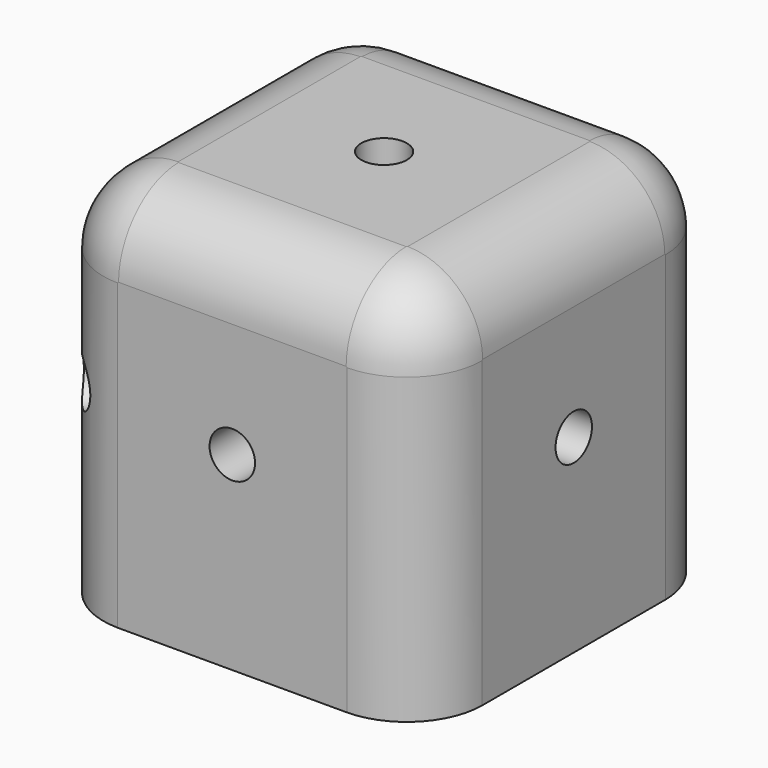
from build123d import *

# Parameters (mm, degrees)
F0_W         = 25
F0_H         = 25
F1_DEPTH     = 12.5
F2_R         = 1.5
F3_DEPTH     = 25
F4_R         = 1.5
F5_DEPTH     = 25.001
F6_R         = 1.5
F7_DEPTH     = 25.001
F8_T1_DEPTH  = 32.5014485681
F8_T3_DEPTH  = 14.9980686292
F8_T5_DEPTH  = 14.9980686292
F8_S9_W      = 5.5015022539
F8_S9_H      = 5.5015022539
F8_T10_DEPTH = 5.501502254
F8_S15_W     = 5.5015022539
F8_S15_H     = 5.5015022539
F8_T16_DEPTH = 5.501502254
F8_S21_W     = 5.5015022539
F8_S21_H     = 5.5015022539
F8_T22_DEPTH = 5.501502254
F8_S27_W     = 5.5015022539
F8_S27_H     = 5.5015022539
F8_T28_DEPTH = 5.501502254
F10_R        = 1.5
F11_DEPTH    = 31.8208051534
F13_R        = 1.5
F14_DEPTH    = 31.8208052241


# Not quite as in the source:
# - a fillet or chamfer that OpenCascade refuses, or shapes differently, is made with other operations: its cross-section is extruded or revolved along the edge and cut away or added


with BuildPart() as f1:
    # F0 (on Front) → F1 (new body, symmetric)
    with BuildSketch(Plane.XZ):
        Rectangle(F0_W, F0_H)
    extrude(amount=F1_DEPTH, both=True)

    # F2 (on face) → F3 (cut, through all)
    with BuildSketch(Plane.XZ.offset(12.5)):
        Circle(F2_R)
    extrude(amount=-F3_DEPTH, mode=Mode.SUBTRACT)

    # F4 (on face) → F5 (cut, through all)
    with BuildSketch(Plane(origin=(0, 0, -12.5), x_dir=(1, 0, 0), z_dir=(0, 0, -1))):
        Circle(F4_R)
    extrude(amount=-F5_DEPTH, mode=Mode.SUBTRACT)

    # F6 (on face) → F7 (cut, through all)
    with BuildSketch(Plane(origin=(-12.5, 0, 0), x_dir=(0, -1, 0), z_dir=(-1, 0, 0))):
        Circle(F6_R)
    extrude(amount=-F7_DEPTH, mode=Mode.SUBTRACT)

    # F8: fillet of radius 5 on 8 edges, made by hand

    # F8_s2 → F8_t1 (cut)
    with BuildSketch(Plane.XY.offset(-25.0024142536)):
        with BuildLine():
            ThreePointArc((7.4990343146, -12.5004), (11.0355339059, -11.0355339059), (12.5004, -7.4990343146))
            Line((12.5004, -7.4990343146), (13.0005365685, -7.4990343146))
            ThreePointArc((13.0005365685, -7.4990343146), (13.0001365685, -9.9995171573), (13.0001365685, -12.5))
            Line((13.0001365685, -12.5), (12.5, -13.0001365685))
            ThreePointArc((12.5, -13.0001365685), (9.9995171573, -13.0001365685), (7.4990343146, -13.0005365685))
            Line((7.4990343146, -13.0005365685), (7.4990343146, -12.5004))
        make_face()
        with BuildLine():
            ThreePointArc((-12.5004, 7.4990343146), (-11.0355339059, 11.0355339059), (-7.4990343146, 12.5004))
            Line((-7.4990343146, 12.5004), (-7.4990343146, 13.0005365685))
            ThreePointArc((-7.4990343146, 13.0005365685), (-9.9995171573, 13.0001365685), (-12.5, 13.0001365685))
            Line((-12.5, 13.0001365685), (-13.0001365685, 12.5))
            ThreePointArc((-13.0001365685, 12.5), (-13.0001365685, 9.9995171573), (-13.0005365685, 7.4990343146))
            Line((-13.0005365685, 7.4990343146), (-12.5004, 7.4990343146))
        make_face()
        with BuildLine():
            ThreePointArc((-12.5004, -7.4990343146), (-11.0355339059, -11.0355339059), (-7.4990343146, -12.5004))
            Line((-7.4990343146, -12.5004), (-7.4990343146, -13.0005365685))
            ThreePointArc((-7.4990343146, -13.0005365685), (-9.9995171573, -13.0001365685), (-12.5, -13.0001365685))
            Line((-12.5, -13.0001365685), (-13.0001365685, -12.5))
            ThreePointArc((-13.0001365685, -12.5), (-13.0001365685, -9.9995171573), (-13.0005365685, -7.4990343146))
            Line((-13.0005365685, -7.4990343146), (-12.5004, -7.4990343146))
        make_face()
        with BuildLine():
            ThreePointArc((7.4990343146, 12.5004), (11.0355339059, 11.0355339059), (12.5004, 7.4990343146))
            Line((12.5004, 7.4990343146), (13.0005365685, 7.4990343146))
            ThreePointArc((13.0005365685, 7.4990343146), (13.0001365685, 9.9995171573), (13.0001365685, 12.5))
            Line((13.0001365685, 12.5), (12.5, 13.0001365685))
            ThreePointArc((12.5, 13.0001365685), (9.9995171573, 13.0001365685), (7.4990343146, 13.0005365685))
            Line((7.4990343146, 13.0005365685), (7.4990343146, 12.5004))
        make_face()
    extrude(amount=F8_T1_DEPTH, mode=Mode.SUBTRACT)

    # F8_s4 → F8_t3 (cut)
    with BuildSketch(Plane.XZ.offset(-7.4990343146)):
        with BuildLine():
            ThreePointArc((7.4990343146, 12.5004), (11.0355339059, 11.0355339059), (12.5004, 7.4990343146))
            Line((12.5004, 7.4990343146), (13.0005365685, 7.4990343146))
            ThreePointArc((13.0005365685, 7.4990343146), (13.0001365685, 9.9995171573), (13.0001365685, 12.5))
            Line((13.0001365685, 12.5), (12.5, 13.0001365685))
            ThreePointArc((12.5, 13.0001365685), (9.9995171573, 13.0001365685), (7.4990343146, 13.0005365685))
            Line((7.4990343146, 13.0005365685), (7.4990343146, 12.5004))
        make_face()
        with BuildLine():
            ThreePointArc((-12.5004, 7.4990343146), (-11.0355339059, 11.0355339059), (-7.4990343146, 12.5004))
            Line((-7.4990343146, 12.5004), (-7.4990343146, 13.0005365685))
            ThreePointArc((-7.4990343146, 13.0005365685), (-9.9995171573, 13.0001365685), (-12.5, 13.0001365685))
            Line((-12.5, 13.0001365685), (-13.0001365685, 12.5))
            ThreePointArc((-13.0001365685, 12.5), (-13.0001365685, 9.9995171573), (-13.0005365685, 7.4990343146))
            Line((-13.0005365685, 7.4990343146), (-12.5004, 7.4990343146))
        make_face()
    extrude(amount=F8_T3_DEPTH, mode=Mode.SUBTRACT)

    # F8_s6 → F8_t5 (cut)
    with BuildSketch(Plane.YZ.offset(-7.4990343146)):
        with BuildLine():
            ThreePointArc((12.5004, 7.4990343146), (11.0355339059, 11.0355339059), (7.4990343146, 12.5004))
            Line((7.4990343146, 12.5004), (7.4990343146, 13.0005365685))
            ThreePointArc((7.4990343146, 13.0005365685), (9.9995171573, 13.0001365685), (12.5, 13.0001365685))
            Line((12.5, 13.0001365685), (13.0001365685, 12.5))
            ThreePointArc((13.0001365685, 12.5), (13.0001365685, 9.9995171573), (13.0005365685, 7.4990343146))
            Line((13.0005365685, 7.4990343146), (12.5004, 7.4990343146))
        make_face()
        with BuildLine():
            ThreePointArc((-7.4990343146, 12.5004), (-11.0355339059, 11.0355339059), (-12.5004, 7.4990343146))
            Line((-12.5004, 7.4990343146), (-13.0005365685, 7.4990343146))
            ThreePointArc((-13.0005365685, 7.4990343146), (-13.0001365685, 9.9995171573), (-13.0001365685, 12.5))
            Line((-13.0001365685, 12.5), (-12.5, 13.0001365685))
            ThreePointArc((-12.5, 13.0001365685), (-9.9995171573, 13.0001365685), (-7.4990343146, 13.0005365685))
            Line((-7.4990343146, 13.0005365685), (-7.4990343146, 12.5004))
        make_face()
    extrude(amount=F8_T5_DEPTH, mode=Mode.SUBTRACT)


with BuildPart() as f8_tool8:
    # F8_s9 → F8_t10 (new body)
    with BuildSketch(Plane.XY.offset(7.4990343146)):
        with Locations((10.2497854415, -10.2497854415)):
            Rectangle(F8_S9_W, F8_S9_H)
    extrude(amount=F8_T10_DEPTH)

    # F8_s11 → F8_t12 (revolve, cut)
    with BuildSketch(Plane(origin=(7.4990343146, -7.4990343146, 7.4990343146), x_dir=(-0.7071067812, 0.7071067812, 0), z_dir=(0.7071067812, 0.7071067812, 0))):
        with BuildLine():
            ThreePointArc((0, -5.0013656854), (5.0013656854, 0), (0, 5.0013656854))
            Line((0, 5.0013656854), (0, -5.0013656854))
        make_face()
    revolve(axis=Axis((7.4990343146, -7.4990343146, 7.4990343146), (0, 0, 1)), mode=Mode.SUBTRACT)


with BuildPart() as f1_1:
    add(f1.part)

    # F8_t7: cut F8_tool8
    add(f8_tool8.part, mode=Mode.SUBTRACT)


with BuildPart() as f8_tool14:
    # F8_s15 → F8_t16 (new body)
    with BuildSketch(Plane.XZ.offset(-7.4990343146)):
        with Locations((10.2497854415, 10.2497854415)):
            Rectangle(F8_S15_W, F8_S15_H)
    extrude(amount=-F8_T16_DEPTH)

    # F8_s17 → F8_t18 (revolve, cut)
    with BuildSketch(Plane(origin=(7.4990343146, 7.4990343146, 7.4990343146), x_dir=(-0.7071067812, 0, -0.7071067812), z_dir=(0.7071067812, 0, -0.7071067812))):
        with BuildLine():
            ThreePointArc((0, -5.0013656854), (5.0013656854, 0), (0, 5.0013656854))
            Line((0, 5.0013656854), (0, -5.0013656854))
        make_face()
    revolve(axis=Axis((7.4990343146, 7.4990343146, 7.4990343146), (0, 1, 0)), mode=Mode.SUBTRACT)


with BuildPart() as f1_2:
    add(f1_1.part)

    # F8_t13: cut F8_tool14
    add(f8_tool14.part, mode=Mode.SUBTRACT)


with BuildPart() as f8_tool20:
    # F8_s21 → F8_t22 (new body)
    with BuildSketch(Plane.YZ.offset(-7.4990343146)):
        with Locations((10.2497854415, 10.2497854415)):
            Rectangle(F8_S21_W, F8_S21_H)
    extrude(amount=-F8_T22_DEPTH)

    # F8_s23 → F8_t24 (revolve, cut)
    with BuildSketch(Plane(origin=(-7.4990343146, 7.4990343146, 7.4990343146), x_dir=(0, -0.7071067812, -0.7071067812), z_dir=(0, 0.7071067812, -0.7071067812))):
        with BuildLine():
            ThreePointArc((0, -5.0013656854), (5.0013656854, 0), (0, 5.0013656854))
            Line((0, 5.0013656854), (0, -5.0013656854))
        make_face()
    revolve(axis=Axis((-7.4990343146, 7.4990343146, 7.4990343146), (-1, 0, 0)), mode=Mode.SUBTRACT)


with BuildPart() as f1_3:
    add(f1_2.part)

    # F8_t19: cut F8_tool20
    add(f8_tool20.part, mode=Mode.SUBTRACT)


with BuildPart() as f8_tool26:
    # F8_s27 → F8_t28 (new body)
    with BuildSketch(Plane.YZ.offset(-7.4990343146)):
        with Locations((-10.2497854415, 10.2497854415)):
            Rectangle(F8_S27_W, F8_S27_H)
    extrude(amount=-F8_T28_DEPTH)

    # F8_s29 → F8_t30 (revolve, cut)
    with BuildSketch(Plane(origin=(-7.4990343146, -7.4990343146, 7.4990343146), x_dir=(0, 0.7071067812, -0.7071067812), z_dir=(0, 0.7071067812, 0.7071067812))):
        with BuildLine():
            ThreePointArc((0, -5.0013656854), (5.0013656854, 0), (0, 5.0013656854))
            Line((0, 5.0013656854), (0, -5.0013656854))
        make_face()
    revolve(axis=Axis((-7.4990343146, -7.4990343146, 7.4990343146), (-1, 0, 0)), mode=Mode.SUBTRACT)


with BuildPart() as f1_4:
    add(f1_3.part)

    # F8_t25: cut F8_tool26
    add(f8_tool26.part, mode=Mode.SUBTRACT)

    # F10 (on face) → F11 (cut, through all)
    with BuildSketch(Plane(origin=(10, 10, 0), x_dir=(-0.7071067812, 0.7071067812, 0), z_dir=(0.7071067812, 0.7071067812, 0))):
        Circle(F10_R)
    extrude(amount=-F11_DEPTH, mode=Mode.SUBTRACT)

    # F13 (on face) → F14 (cut, through all)
    with BuildSketch(Plane(origin=(10, -10, 0), x_dir=(0.7071067812, 0.7071067812, 0), z_dir=(0.7071067812, -0.7071067812, 0))):
        Circle(F13_R)
    extrude(amount=-F14_DEPTH, mode=Mode.SUBTRACT)


solid = f1_4.part
